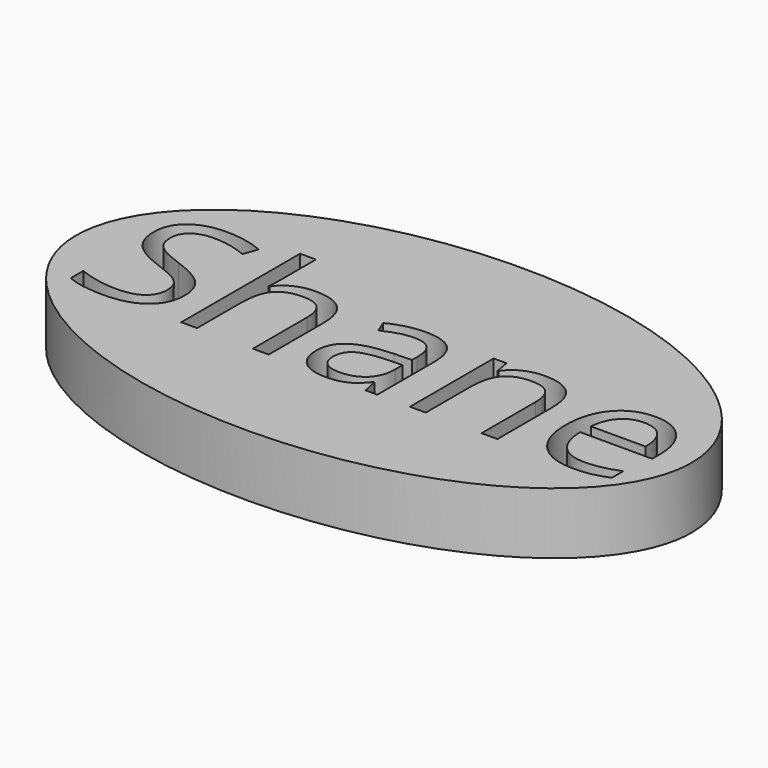
from build123d import *

# Parameters (mm, degrees)
F1_DEPTH     = 7.62
F2_TEXT_SIZE = 24.202072786
F3_DEPTH     = 5.08


# Not quite as in the source:
# - Text() gives the source's letters only with a copy of the font that has no kerning and outlines rounded to 1/6400 em; it was checked with that copy


with BuildPart() as f1:
    # F0 (on Top) → F1 (new body)
    with BuildSketch(Plane.XY):
        with BuildLine():
            add(Edge.make_bspline(
                [(38.1, 0), (38.1, 37.3949769354), (-19.05, 18.6974884677), (-76.2, 0), (-19.05, -18.6974884677), (38.1, -37.3949769354), (38.1, 0)],
                knots=[0, 0, 0, 2.0943951024, 2.0943951024, 4.1887902048, 4.1887902048, 6.2831853072, 6.2831853072, 6.2831853072], degree=2, weights=[1, 0.5, 1, 0.5, 1, 0.5, 1]))
        make_face()
    extrude(amount=F1_DEPTH)

    # F2 (on face) → F3 (cut)
    with BuildSketch(Plane.XY.offset(7.62)):
        with Locations((-34.1671452447, -7.8722220116)):
            Text('Shane', F2_TEXT_SIZE, font='Open Sans', text_align=(TextAlign.LEFT, TextAlign.BOTTOM))
    extrude(amount=-F3_DEPTH, mode=Mode.SUBTRACT)


solid = f1.part
